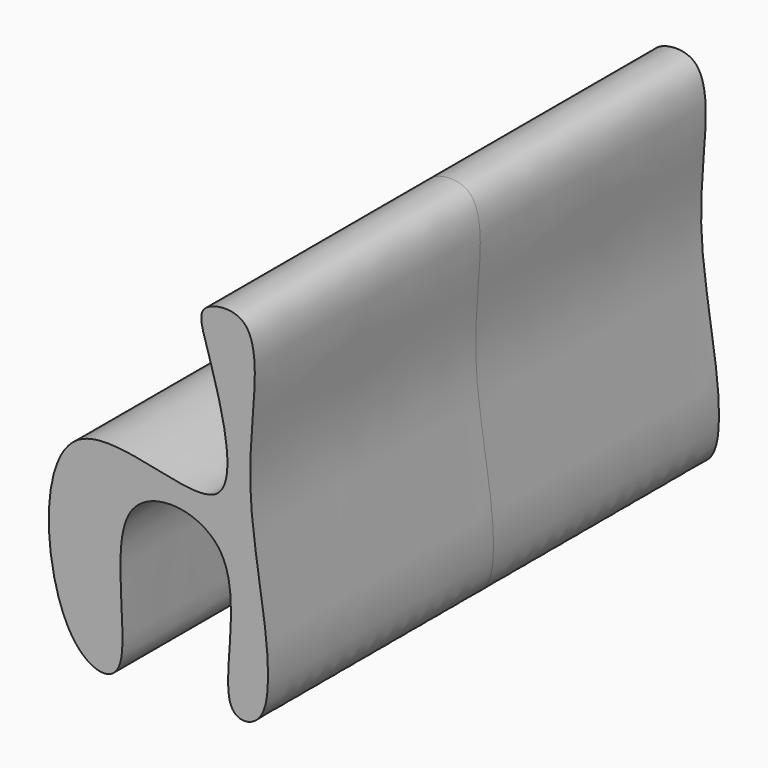
from build123d import *

# Parameters (mm, degrees)
F1_DEPTH = 83


# Not quite as in the source:
# - a feature of the source that left no trace in its solid (it failed there, or was rolled back) is left out
# - the program builds the solid bodies; features that only make, move or delete a surface that nothing else refers to are left out


with BuildPart() as f1:
    # F0 (on Front) → F1 (new body)
    with BuildSketch(Plane.XZ):
        with BuildLine():
            add(Edge.make_bspline(
                [(44.4153994322, 30.5418260396), (43.5974151636, 20.3086251278), (42.6507840735, 3.2423018665), (54.1407203443, -48.3949771722), (31.1439468171, -50.4210964492), (47.787140915, -0.0033898874), (-4.3186889453, 4.8024910331), (13.1777786352, -53.8027179188), (-15.8640972232, -47.7190308224), (-21.5535556267, 29.0399609787), (47.7666049841, -9.5518281776), (30.9136982282, 44.668110771), (27.499697264, 55.8319029277), (46.8889643292, 58.3678169333), (45.1452218553, 39.6720987999), (44.4153994322, 30.5418260396)],
                knots=[0, 0, 0, 0, 0.0813237495, 0.1812831869, 0.2234358388, 0.3161152306, 0.3915195151, 0.4877013808, 0.541589564, 0.6478155404, 0.7419510137, 0.8312586897, 0.8786845551, 0.9274412746, 1, 1, 1, 1], degree=3))
        make_face()
    extrude(amount=F1_DEPTH)

    # F5: F1 across plane


with BuildPart() as f1_1:
    add(f1.part)
    add(f1.part.mirror(Plane.XZ.offset(83)))


solid = f1_1.part
